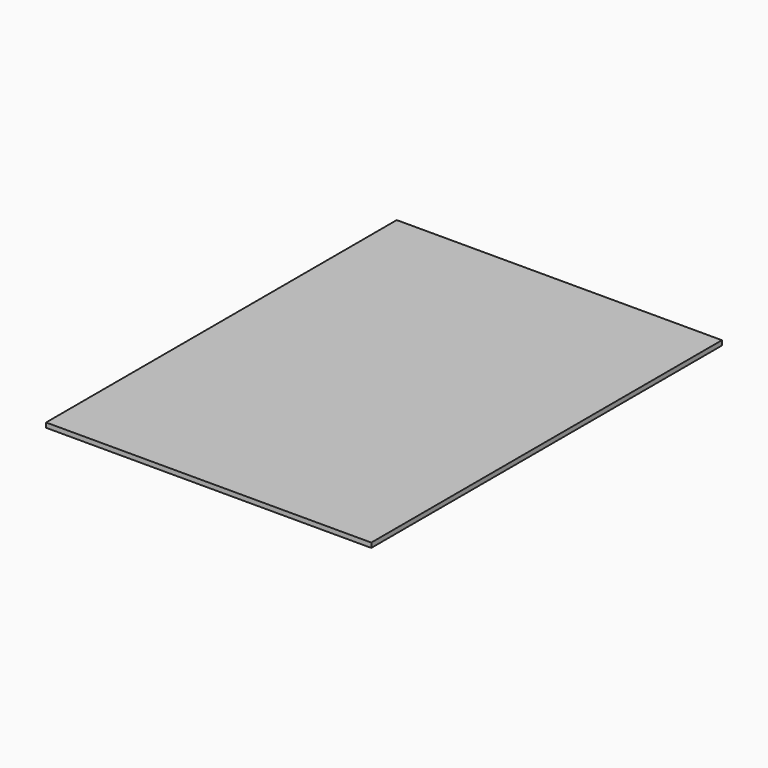
from build123d import *

# Parameters (mm, degrees)
F0_W     = 219.075
F0_H     = 295.275
F1_DEPTH = 3.175


# Not quite as in the source:
# - a length typed as a fraction of an inch, garbled in the dataset ("3 / 203.2 mm" for 3/8 in), is restored


with BuildPart() as f1:
    # F0 (on Top) → F1 (new body)
    with BuildSketch(Plane.XY):
        Rectangle(F0_W, F0_H)
    extrude(amount=F1_DEPTH)


solid = f1.part
